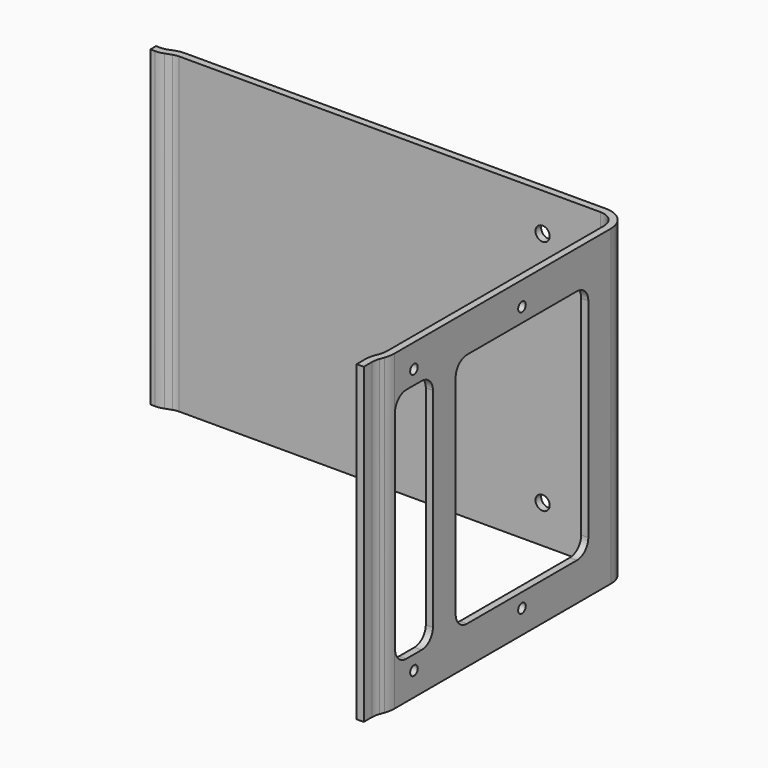
from build123d import *

# Parameters (mm, degrees)
F1_DEPTH  = 66
F2_R      = 1.5
F3_DEPTH  = 25
F4_R      = 1
F5_DEPTH  = 25
F6_R      = 5
F7_R      = 6.5
F8_W      = 11.5
F8_H      = 48
F9_DEPTH  = 100
F11_DEPTH = 66


# Not quite as in the source:
# - a feature names something its author has since deleted; it is built from what else it names


with BuildPart() as f1:
    # F0 (on Top) → F1 (new body)
    with BuildSketch(Plane.XY):
        with BuildLine():
            Line((54.5, 33), (54.5, -24.9880321095))
            Line((54.5, -24.9880321095), (53.5, -27.7355095289))
            Line((53.5, -27.7355095289), (53.5, -31))
            Line((53.5, -31), (55, -31))
            Line((55, -31), (55, -28))
            Line((55, -28), (56, -25.2525225805))
            Line((56, -25.2525225805), (56, 33))
            ThreePointArc((56, 33), (54.5355339059, 36.5355339059), (51, 38))
            Line((51, 38), (-42.5, 38))
            ThreePointArc((-42.5, 38), (-46.0355339059, 36.5355339059), (-47.5, 33))
            Line((-47.5, 33), (-47.5, 0))
            Line((-47.5, 0), (-46.000000001, 0))
            Line((-46.000000001, 0), (-46.000000001, 33))
            ThreePointArc((-46.000000001, 33), (-44.9748737349, 35.4748737349), (-42.5, 36.500000001))
            Line((-42.5, 36.5), (51, 36.5))
            ThreePointArc((51, 36.5), (53.4748737342, 35.4748737342), (54.5, 33))
        make_face()
    extrude(amount=F1_DEPTH)

    # F2 (on face) → F3 (cut)
    with BuildSketch(Plane(origin=(0, 38, 0), x_dir=(-1, 0, 0), z_dir=(0, 1, 0))):
        with Locations((-38.75, 58)):
            Circle(F2_R)
        with Locations((-38.75, 8)):
            Circle(F2_R)
    extrude(amount=-F3_DEPTH, mode=Mode.SUBTRACT)

    # F4 (on face) → F5 (cut)
    with BuildSketch(Plane.YZ.offset(56)):
        with BuildLine():
            Line((-17, 58), (-21, 58))
            ThreePointArc((-21, 58), (-23.1213203436, 57.1213203436), (-24, 55))
            Line((-24, 55), (-24, 11))
            ThreePointArc((-24, 11), (-23.1213203436, 8.8786796564), (-21, 8))
            Line((-21, 8), (-17, 8))
            ThreePointArc((-17, 8), (-14.8786796564, 8.8786796564), (-14, 11))
            Line((-14, 11), (-14, 55))
            ThreePointArc((-14, 55), (-14.8786796564, 57.1213203436), (-17, 58))
        make_face()
        with BuildLine():
            Line((24, 58), (-5, 58))
            ThreePointArc((-5, 58), (-7.1213203436, 57.1213203436), (-8, 55))
            Line((-8, 55), (-8, 11))
            ThreePointArc((-8, 11), (-7.1213203436, 8.8786796564), (-5, 8))
            Line((-5, 8), (24, 8))
            ThreePointArc((24, 8), (26.1213203436, 8.8786796564), (27, 11))
            Line((27, 11), (27, 55))
            ThreePointArc((27, 55), (26.1213203436, 57.1213203436), (24, 58))
        make_face()
        with Locations((-19, 61)):
            Circle(F4_R)
        with Locations((9.5, 61)):
            Circle(F4_R)
        with Locations((9.5, 5)):
            Circle(F4_R)
        with Locations((-19, 5)):
            Circle(F4_R)
    extrude(amount=-F5_DEPTH, mode=Mode.SUBTRACT)

    # F6
    f6_edges = [f1.edges().sort_by_distance(p)[0] for p in [
        (55, -28, 33),
        (54.5, -24.988032, 33),
    ]]
    fillet(f6_edges, radius=F6_R)

    # F7
    f7_edges = [f1.edges().sort_by_distance(p)[0] for p in [
        (56, -25.252523, 33),
        (53.5, -27.73551, 33),
    ]]
    fillet(f7_edges, radius=F7_R)

    # F8 (on Top) → F9 (cut)
    with BuildSketch(Plane.XY):
        with Locations((-43.75, 19)):
            Rectangle(F8_W, F8_H)
    extrude(amount=F9_DEPTH, mode=Mode.SUBTRACT)

    # F10 (on Top) → F11 (join)
    with BuildSketch(Plane.XY):
        with BuildLine():
            Line((-43.2462567555, 37), (-43.2462567555, 35.5))
            Line((-43.2462567555, 35.5), (-42.2462567555, 35.5))
            ThreePointArc((-42.2462567555, 35.5), (-41.3780158671, 35.5759612349), (-40.5361560388, 35.8015368961))
            Line((-40.5361560388, 35.8015368961), (-39.1970705016, 36.2889241728))
            ThreePointArc((-39.1970705016, 36.2889241728), (-38.6077686218, 36.4468271355), (-38, 36.5))
            Line((-38, 36.5), (-38, 38))
            ThreePointArc((-38, 38), (-38.8682408883, 37.9240387651), (-39.7101007166, 37.6984631039))
            Line((-39.7101007166, 37.6984631039), (-41.0491862538, 37.2110758272))
            ThreePointArc((-41.0491862538, 37.2110758272), (-41.6384881336, 37.0531728645), (-42.2462567555, 37))
            Line((-42.2462567555, 37), (-43.2462567555, 37))
        make_face()
    extrude(amount=F11_DEPTH)


solid = f1.part
